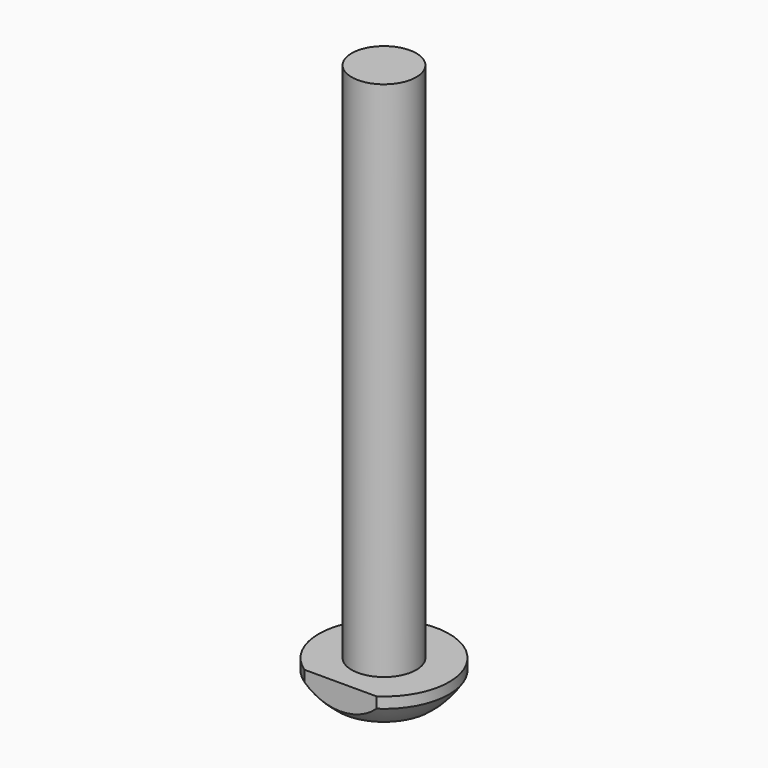
from build123d import *

# Parameters (mm, degrees)
F3_DEPTH = 4.7625


# Not quite as in the source:
# - a length typed as a fraction of an inch, garbled in the dataset ("3 / 203.2 mm" for 3/8 in), is restored


with BuildPart() as f1:
    # F0 (on Front) → F1 (revolve)
    with BuildSketch(Plane.XZ):
        with BuildLine():
            Line((0, 76.2), (0, 0))
            Line((0, 0), (0, -4.7625))
            Line((0, -4.7625), (6.655733594, -4.7625))
            ThreePointArc((6.655733594, -4.7625), (8.2446462119, -3.314423226), (9.525, -1.5875))
            Line((9.525, -1.5875), (9.525, 0))
            Line((9.525, 0), (4.7244, 0))
            Line((4.7244, 0), (4.7244, 76.2))
            Line((4.7244, 76.2), (0, 76.2))
        make_face()
    revolve(axis=Axis((0, 0, 38.1), (0, 0, 1)))

    # F2 (on face) → F3 (cut)
    with BuildSketch(Plane(origin=(0, 0, -4.7625), x_dir=(1, 0, 0), z_dir=(0, 0, -1))):
        with BuildLine():
            Line((0, 7.9375), (5.2651418547, 7.9375))
            ThreePointArc((5.2651418547, 7.9375), (0, 9.525), (-5.2651418547, 7.9375))
            Line((-5.2651418547, 7.9375), (0, 7.9375))
        make_face()
    extrude(amount=-F3_DEPTH, mode=Mode.SUBTRACT)


solid = f1.part
